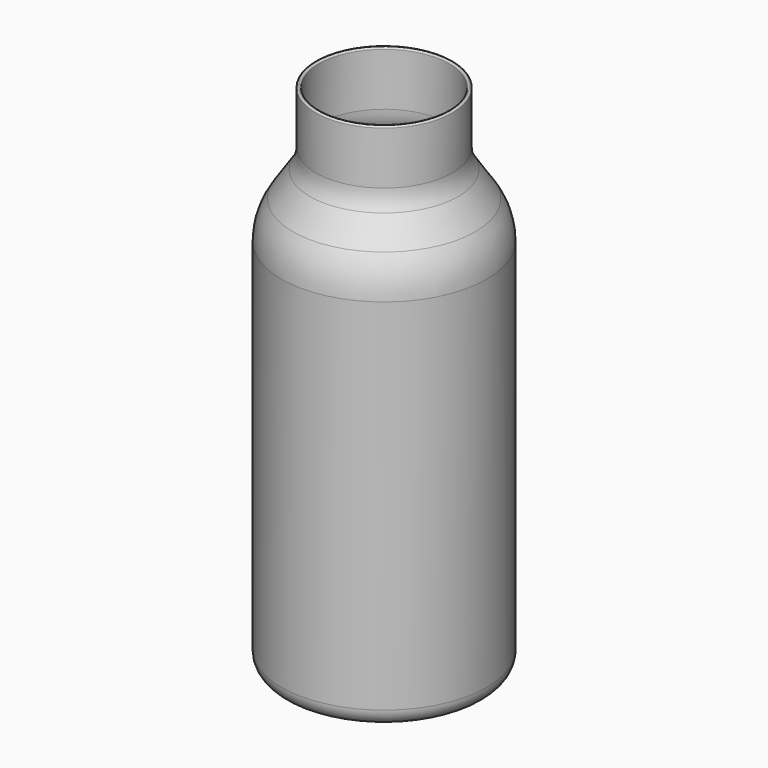
from build123d import *

# Parameters (mm, degrees)
F2_R = 1.26999


# Not quite as in the source:
# - a fillet or chamfer is up to 0.001 mm smaller than in the source, because OpenCascade refuses the exact size


with BuildPart() as f1:
    # F0 (on Front) → F1 (revolve)
    with BuildSketch(Plane.XZ):
        with BuildLine():
            Line((76.2, 12.7), (76.2, 279.4))
            ThreePointArc((76.2, 279.4), (74.0202749456, 294.1210347534), (67.6681549524, 307.5787699682))
            Line((67.6681549524, 307.5787699682), (55.0659225238, 326.4821186111))
            ThreePointArc((55.0659225238, 326.4821186111), (51.8898625272, 333.2109862185), (50.8, 340.5715035952))
            Line((50.8, 340.5715035952), (50.8, 381))
            Line((50.8, 381), (48.26, 381))
            Line((48.26, 381), (48.26, 340.5715035952))
            ThreePointArc((48.26, 340.5715035952), (49.4588487799, 332.4749344808), (52.9525147762, 325.0731801126))
            Line((52.9525147762, 325.0731801126), (65.5547472047, 306.1698314698))
            ThreePointArc((65.5547472047, 306.1698314698), (71.5892611984, 293.3849830157), (73.66, 279.4))
            Line((73.66, 279.4), (73.66, 12.7))
            ThreePointArc((73.66, 12.7), (70.6842048969, 5.5157951031), (63.5, 2.54))
            Line((63.5, 2.54), (0, 2.54))
            Line((0, 2.54), (0, 0))
            Line((0, 0), (63.5, 0))
            ThreePointArc((63.5, 0), (72.4802561211, 3.7197438789), (76.2, 12.7))
        make_face()
    revolve(axis=Axis((0, 0, 199.2018222809), (0, 0, 1)))

    # F2 (radius 1.27 in the source; OpenCascade refuses exactly that, so slightly less here)
    f2_edges = [f1.edges().sort_by_distance(p)[0] for p in [
        (-50.8, 0, 381),
        (-48.26, 0, 381),
    ]]
    fillet(f2_edges, radius=F2_R)


solid = f1.part
